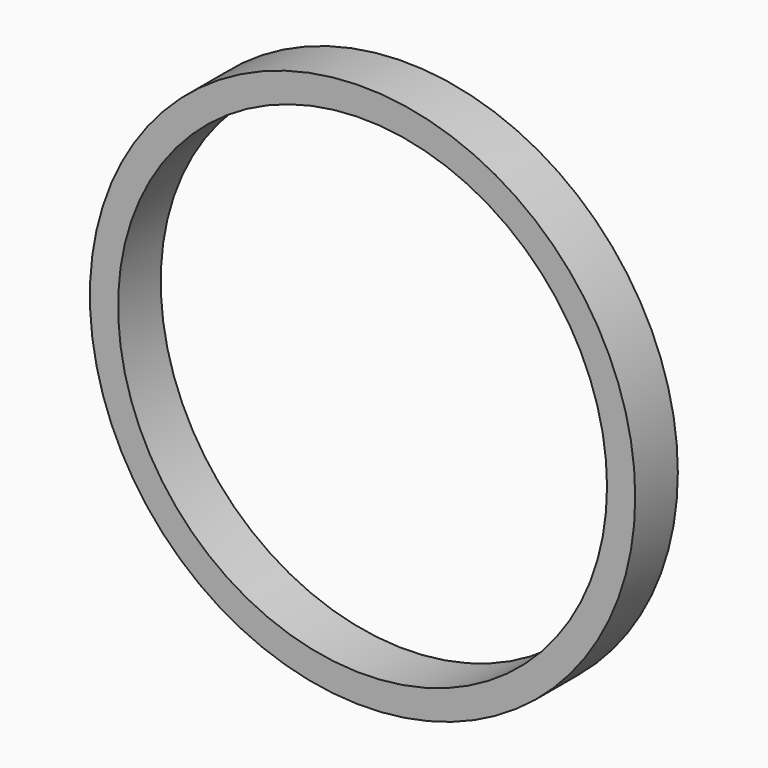
from build123d import *

# Parameters (mm, degrees)
F0_R     = 25.04
F0_R_2   = 22.45
F1_DEPTH = 2.446


# Not quite as in the source:
# - a feature of the source that left no trace in its solid (it failed there, or was rolled back) is left out


with BuildPart() as f1:
    # F0 (on Front) → F1 (new body, symmetric)
    with BuildSketch(Plane.XZ):
        Circle(F0_R)
        Circle(F0_R_2, mode=Mode.SUBTRACT)
    extrude(amount=F1_DEPTH, both=True)


solid = f1.part
